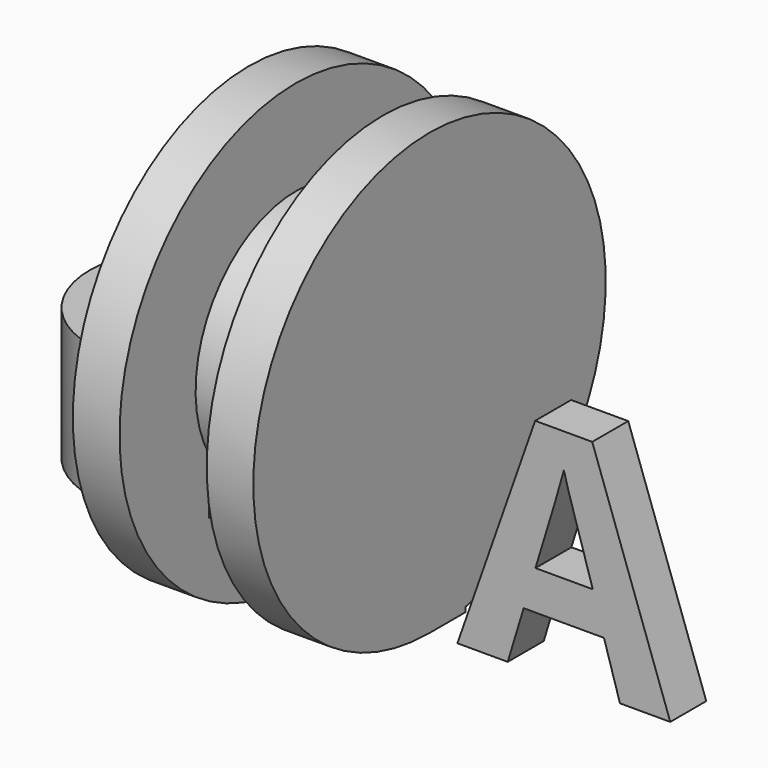
from build123d import *

# Parameters (mm, degrees)
F0_TEXT_SIZE = 174.113145719
F1_DEPTH     = 25.4
F2_R         = 57.382576072
F4_DEPTH     = 74.93


# Not quite as in the source:
# - Text() gives the source's letters only with a copy of the font that has no kerning and outlines rounded to 1/6400 em; it was checked with that copy


with BuildPart() as f1:
    # F0 (on Front) → F1 (new body)
    with BuildSketch(Plane.XZ):
        with Locations((-101.1925041676, -57.4374347925)):
            Text('HA', F0_TEXT_SIZE, font='Open Sans', font_style=FontStyle.BOLD, text_align=(TextAlign.LEFT, TextAlign.BOTTOM))
    extrude(amount=F1_DEPTH)

    # F1_face (on face) → F3 (revolve)
    with BuildSketch(Plane(origin=(-34.6484033894, -25.4, 5.0613552799), x_dir=(1, 0, 0), z_dir=(0, -1, 0))):
        Polygon((24.6748644712, -62.4987900724), (50.9550674031, -62.4987900724), (50.9550674031, 61.8016728635), (24.6748644712, 61.8016728635), (24.6748644712, 13.0771972412), (-24.5393043735, 13.0771972412), (-24.5393043735, 61.8016728635), (-50.9011228425, 61.8016728635), (-50.9011228425, -62.4987900724), (-24.5393043735, -62.4987900724), (-24.5393043735, -8.8501770478), (24.6748644712, -8.8501770478), align=None)
    revolve(axis=Axis((-72.3686169974, -25.4, 66.8630281434), (1, 0, 0)))

    # F2 (on Top) → F4 (join)
    with BuildSketch(Plane.XY):
        with Locations((-100.7193699479, -46.8817055225)):
            Circle(F2_R)
    extrude(amount=F4_DEPTH)


solid = f1.part
